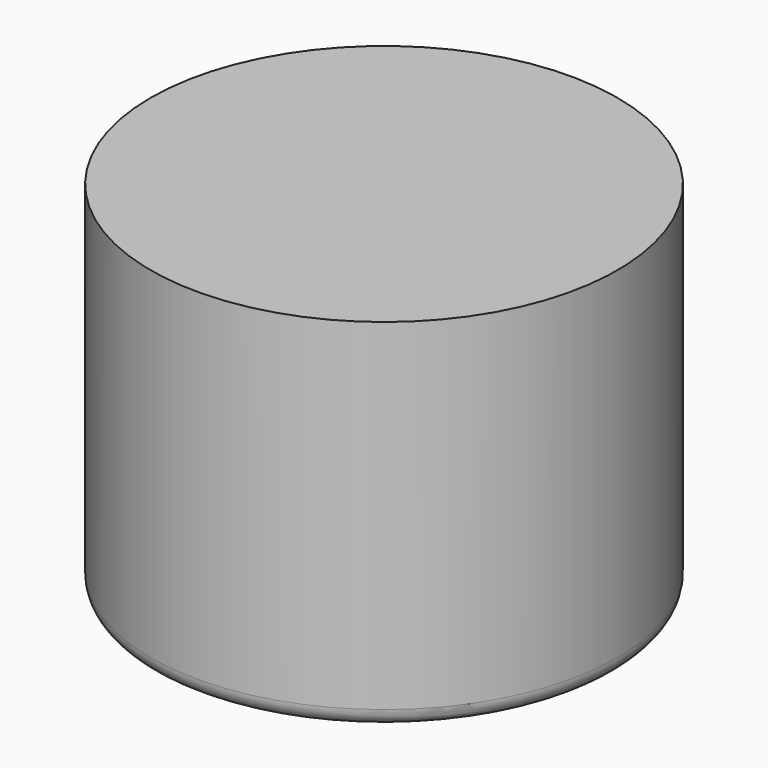
from build123d import *

# Parameters (mm, degrees)
F2_R = 0.5
F3_R = 0.99999


# Not quite as in the source:
# - a fillet or chamfer is up to 0.001 mm smaller than in the source, because OpenCascade refuses the exact size


with BuildPart() as f1:
    # F0 (on Front) → F1 (revolve)
    with BuildSketch(Plane.XZ):
        Polygon((7.9903845042, 17.1442301405), (-5.0096154958, 17.1442301405), (-5.0096154958, -2.8557698595), (-3.0096154958, -2.8557698595), (-3.0096154958, 15.1442301405), (7.9903845042, 15.1442301405), align=None)
    revolve(axis=Axis((7.9903845042, 0, 16.1442301405), (0, 0, -1)))

    # F2
    f2_edges = [f1.edges().sort_by_distance(p)[0] for p in [
        (18.990385, 0, 15.14423),
    ]]
    fillet(f2_edges, radius=F2_R)

    # F3 (radius 1 in the source; OpenCascade refuses exactly that, so slightly less here)
    f3_edges = [f1.edges().sort_by_distance(p)[0] for p in [
        (20.990385, 0, -2.85577),
        (18.990385, 0, -2.85577),
    ]]
    fillet(f3_edges, radius=F3_R)


solid = f1.part
